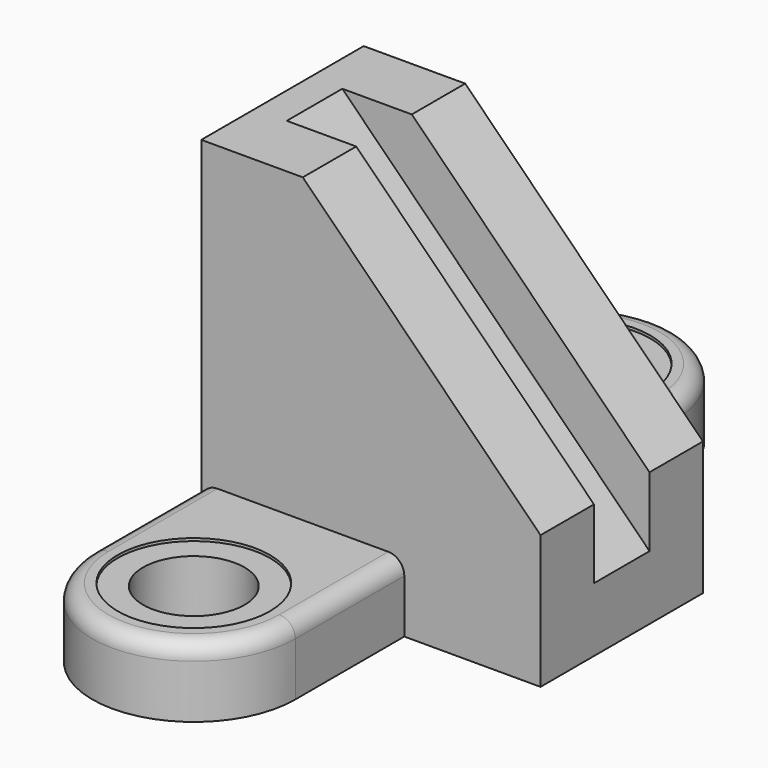
from build123d import *

# Parameters (mm, degrees)
F1_DEPTH  = 26
F5_DEPTH  = 76
F8_DEPTH  = 26
F9_R      = 28.5
F10_DEPTH = 1
F11_R     = 19
F12_DEPTH = 25
F13_R     = 6


# Not quite as in the source:
# - a pattern or mirror of a feature is missing from the dataset's text; its kind, count and spacing are read off the source's solid


with BuildPart() as f1:
    # F0 (on Top) → F1 (new body)
    with BuildSketch(Plane.XY):
        with BuildLine():
            Line((38, -89), (38, 89))
            ThreePointArc((38, 89), (0, 127), (-38, 89))
            Line((-38, 89), (-38, -89))
            ThreePointArc((-38, -89), (0, -127), (38, -89))
        make_face()
    extrude(amount=F1_DEPTH)

    # F4 (on offset) → F5 (join)
    with BuildSketch(Plane.XZ.offset(38)):
        Polygon((-38, 50), (-38, 0), (89, 0), (89, 50), (0, 139), (-38, 139), align=None)
    extrude(amount=-F5_DEPTH)

    # F7 (on offset) → F8 (cut)
    with BuildSketch(Plane.XZ.offset(13)):
        Polygon((89, 50), (0, 139), (-26, 139), (89, 24), align=None)
    extrude(amount=-F8_DEPTH, mode=Mode.SUBTRACT)

    # F9 (on face) → F10 (cut)
    with BuildSketch(Plane.XY.offset(26)):
        with Locations((0, 89)):
            Circle(F9_R)
    f10 = extrude(amount=-F10_DEPTH, mode=Mode.SUBTRACT)

    # F10_copies: F10 across plane
    add(f10.mirror(Plane(origin=(0, 0, 0), x_dir=(0, 0, -1), z_dir=(0, -1, 0))), mode=Mode.SUBTRACT)

    # F11 (on face) → F12 (cut, through all)
    with BuildSketch(Plane.XY.offset(25)):
        with Locations((0, 89)):
            Circle(F11_R)
    f12 = extrude(amount=-F12_DEPTH, mode=Mode.SUBTRACT)

    # F12_copies: F12 across plane
    add(f12.mirror(Plane(origin=(0, 0, 0), x_dir=(0, 0, -1), z_dir=(0, -1, 0))), mode=Mode.SUBTRACT)

    # F13
    f13_edges = [f1.edges().sort_by_distance(p)[0] for p in [
        (38, -63.5, 26),
        (38, 63.5, 26),
        (0, -127, 26),
        (-38, -63.5, 26),
        (-38, 63.5, 26),
        (0, 127, 26),
    ]]
    fillet(f13_edges, radius=F13_R)


solid = f1.part
